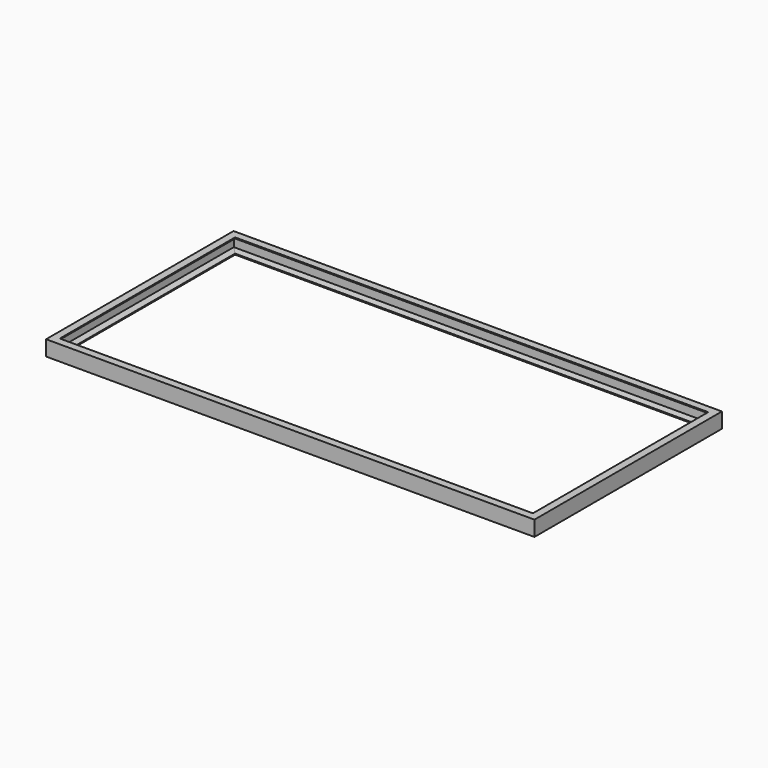
from build123d import *


with BuildPart() as f2:
    # F2: sweep along a path in F0
    with BuildLine(Plane.XY) as f2_path:
        Line((0, 0), (2438.4, 0))
        Line((2438.4, 0), (2438.4, 1170))
        Line((2438.4, 1170), (0, 1170))
        Line((0, 1170), (0, 0))
    # F1 (on Right) → F2 (sweep)
    with BuildSketch(Plane.YZ):
        Polygon((38.1, 0), (0, 0), (0, -76.2), (38.1, -76.2), (38.1, -71.12), (6.35, -66.2), (6.35, -10), (38.1, -5.08), align=None)
    sweep(path=f2_path.line, transition=Transition.RIGHT)


solid = f2.part
